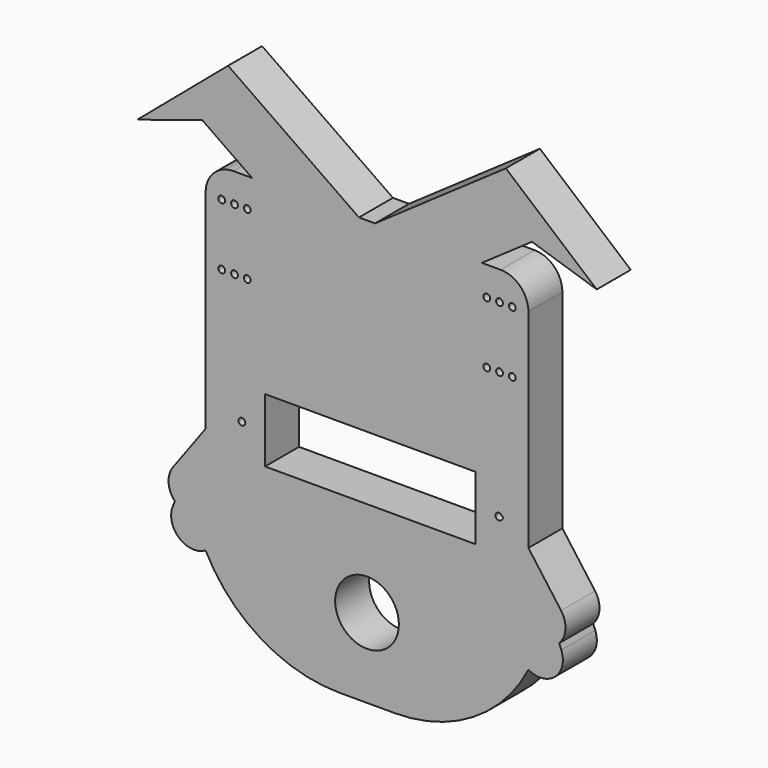
from build123d import *

# Parameters (mm, degrees)
F0_R        = 15
F0_R_2      = 1.6
F1_DEPTH    = 20
F2_R        = 11.6045153918
F3_DEPTH    = 20
F4_T1_DEPTH = 334.7254047122
F6_R        = 13.1169251871
F7_T1_DEPTH = 119.353153646
F7_T3_DEPTH = 204.1085089788


# Not quite as in the source:
# - a fillet or chamfer that OpenCascade refuses, or shapes differently, is made with other operations: its cross-section is extruded or revolved along the edge and cut away or added


with BuildPart() as f1:
    # F0 (on Front) → F1 (new body)
    with BuildSketch(Plane.XZ):
        Polygon((-54.1030839086, 102.6), (-76.0052064898, 102.6), (-76.0052064898, -8.4487323015), (-76.0052064898, -58.9213789776), (-76.0052064898, -97.4), (75.9947935102, -97.4), (75.9947935102, -58.9213789776), (75.9947935102, -8.4487323015), (75.9947935102, 102.6), (54.0926709289, 102.6), (3.7848638975, 102.6), (-0.0052064898, 102.6), (-3.7952768771, 102.6), align=None)
        with Locations((0, -60)):
            Circle(F0_R, mode=Mode.SUBTRACT)
        Polygon((-48.0052064898, 15), (-0.0052064898, 15), (50.9947935102, 15), (63.2902167228, 1.058300535), (64.2235500655, 0), (63.2902167424, -1.0583005129), (50.9947935102, -15), (-48.0052064898, -15), (-61.2339630452, 0), align=None, mode=Mode.SUBTRACT)
        with Locations((-68.4052064898, 60)):
            Circle(F0_R_2, mode=Mode.SUBTRACT)
        with Locations((-62.4052064898, 60)):
            Circle(F0_R_2, mode=Mode.SUBTRACT)
        with Locations((-56.4052064898, 60)):
            Circle(F0_R_2, mode=Mode.SUBTRACT)
        with Locations((-68.4052064898, 89)):
            Circle(F0_R_2, mode=Mode.SUBTRACT)
        with Locations((-62.4052064898, 89)):
            Circle(F0_R_2, mode=Mode.SUBTRACT)
        with Locations((-56.4052064898, 89)):
            Circle(F0_R_2, mode=Mode.SUBTRACT)
        with Locations((56.3947935102, 60)):
            Circle(F0_R_2, mode=Mode.SUBTRACT)
        with Locations((62.3947935102, 60)):
            Circle(F0_R_2, mode=Mode.SUBTRACT)
        with Locations((68.3947935102, 60)):
            Circle(F0_R_2, mode=Mode.SUBTRACT)
        with Locations((56.3947935102, 89)):
            Circle(F0_R_2, mode=Mode.SUBTRACT)
        with Locations((62.3947935102, 89)):
            Circle(F0_R_2, mode=Mode.SUBTRACT)
        with Locations((68.3947935102, 89)):
            Circle(F0_R_2, mode=Mode.SUBTRACT)
        Polygon((-77.668659389, 119.0051808953), (-54.1030839086, 102.6), (-3.7952768771, 102.6), (-65.412312746, 145.4675197601), (-108.1871464849, 109.1671809554), align=None)
        Polygon((-76.0052064898, -58.9213789776), (-76.0052064898, -8.4487323015), (-103.1352177745, -45.4250201583), (-90.5148283129, -43.2038009167), (-105.0179273372, -79.8825249076), align=None)
        Polygon((65.4018997664, 145.4675197601), (3.7848638975, 102.6), (54.0926709289, 102.6), (77.6582464094, 119.0051808953), (108.1767335052, 109.1671809554), align=None)
        Polygon((75.9947935102, -8.4487323015), (75.9947935102, -58.9213789776), (105.0075143576, -79.8825249076), (90.5044153333, -43.2038009167), (103.1248047948, -45.4250201583), align=None)
        with BuildLine():
            Line((63.2902167228, 1.058300535), (50.9947935102, 15))
            Line((50.9947935102, 15), (50.9947935102, -15))
            Line((50.9947935102, -15), (63.2902167424, -1.0583005129))
            ThreePointArc((63.2902167424, -1.0583005129), (60.4902167322, -1.48e-08), (63.2902167228, 1.058300535))
        make_face()
        Polygon((-48.0052064898, -15), (-48.0052064898, 15), (-61.2339630452, 0), align=None)
        with Locations((-58.9281324463, 0)):
            Circle(F0_R_2, mode=Mode.SUBTRACT)
    extrude(amount=F1_DEPTH)

    # F2
    f2_edges = [f1.edges().sort_by_distance(p)[0] for p in [
        (-76.005206, -10, 102.6),
        (-76.005206, -10, -97.4),
        (75.994794, -10, -97.4),
        (75.994794, -10, 102.6),
    ]]
    fillet(f2_edges, radius=F2_R)

    # F0 (on Front) → F3 (join)
    with BuildSketch(Plane.XZ):
        Polygon((-54.1030839086, 102.6), (-76.0052064898, 102.6), (-76.0052064898, -8.4487323015), (-76.0052064898, -58.9213789776), (-76.0052064898, -97.4), (75.9947935102, -97.4), (75.9947935102, -58.9213789776), (75.9947935102, -8.4487323015), (75.9947935102, 102.6), (54.0926709289, 102.6), (3.7848638975, 102.6), (-0.0052064898, 102.6), (-3.7952768771, 102.6), align=None)
        with Locations((0, -60)):
            Circle(F0_R, mode=Mode.SUBTRACT)
        Polygon((-48.0052064898, 15), (-0.0052064898, 15), (50.9947935102, 15), (63.2902167228, 1.058300535), (64.2235500655, 0), (63.2902167424, -1.0583005129), (50.9947935102, -15), (-48.0052064898, -15), (-61.2339630452, 0), align=None, mode=Mode.SUBTRACT)
        with Locations((-68.4052064898, 60)):
            Circle(F0_R_2, mode=Mode.SUBTRACT)
        with Locations((-62.4052064898, 60)):
            Circle(F0_R_2, mode=Mode.SUBTRACT)
        with Locations((-56.4052064898, 60)):
            Circle(F0_R_2, mode=Mode.SUBTRACT)
        with Locations((-68.4052064898, 89)):
            Circle(F0_R_2, mode=Mode.SUBTRACT)
        with Locations((-62.4052064898, 89)):
            Circle(F0_R_2, mode=Mode.SUBTRACT)
        with Locations((-56.4052064898, 89)):
            Circle(F0_R_2, mode=Mode.SUBTRACT)
        with Locations((56.3947935102, 60)):
            Circle(F0_R_2, mode=Mode.SUBTRACT)
        with Locations((62.3947935102, 60)):
            Circle(F0_R_2, mode=Mode.SUBTRACT)
        with Locations((68.3947935102, 60)):
            Circle(F0_R_2, mode=Mode.SUBTRACT)
        with Locations((56.3947935102, 89)):
            Circle(F0_R_2, mode=Mode.SUBTRACT)
        with Locations((62.3947935102, 89)):
            Circle(F0_R_2, mode=Mode.SUBTRACT)
        with Locations((68.3947935102, 89)):
            Circle(F0_R_2, mode=Mode.SUBTRACT)
        Polygon((-77.668659389, 119.0051808953), (-54.1030839086, 102.6), (-3.7952768771, 102.6), (-65.412312746, 145.4675197601), (-108.1871464849, 109.1671809554), align=None)
        Polygon((-76.0052064898, -58.9213789776), (-76.0052064898, -8.4487323015), (-103.1352177745, -45.4250201583), (-90.5148283129, -43.2038009167), (-105.0179273372, -79.8825249076), align=None)
        Polygon((65.4018997664, 145.4675197601), (3.7848638975, 102.6), (54.0926709289, 102.6), (77.6582464094, 119.0051808953), (108.1767335052, 109.1671809554), align=None)
        Polygon((75.9947935102, -8.4487323015), (75.9947935102, -58.9213789776), (105.0075143576, -79.8825249076), (90.5044153333, -43.2038009167), (103.1248047948, -45.4250201583), align=None)
        Polygon((-48.0052064898, -15), (-48.0052064898, 15), (-61.2339630452, 0), align=None)
        with Locations((-58.9281324463, 0)):
            Circle(F0_R_2, mode=Mode.SUBTRACT)
        with BuildLine():
            Line((63.2902167228, 1.058300535), (50.9947935102, 15))
            Line((50.9947935102, 15), (50.9947935102, -15))
            Line((50.9947935102, -15), (63.2902167424, -1.0583005129))
            ThreePointArc((63.2902167424, -1.0583005129), (60.4902167322, -1.48e-08), (63.2902167228, 1.058300535))
        make_face()
    extrude(amount=F3_DEPTH)

    # F4: fillet of radius 70.723525766 on 2 edges, made by hand

    # F4_s2 → F4_t1 (cut)
    with BuildSketch(Plane.XZ.offset(-157.3627023561)):
        with BuildLine():
            ThreePointArc((-76.0052064898, -58.9213789776), (-49.9474116045, -87.018376956), (-13.0601255474, -97.4))
            Line((-13.0601255474, -97.4), (-76.0052064898, -97.4))
            Line((-76.0052064898, -97.4), (-76.0052064898, -58.9213789776))
        make_face()
        with BuildLine():
            ThreePointArc((13.0497125677, -97.4), (49.9369986248, -87.018376956), (75.9947935102, -58.9213789776))
            Line((75.9947935102, -58.9213789776), (75.9947935102, -97.4))
            Line((75.9947935102, -97.4), (13.0497125677, -97.4))
        make_face()
    extrude(amount=F4_T1_DEPTH, mode=Mode.SUBTRACT)

    # F6
    f6_edges = [f1.edges().sort_by_distance(p)[0] for p in [
        (75.994794, -10, 102.6),
        (-76.005206, -10, 102.6),
    ]]
    fillet(f6_edges, radius=F6_R)

    # F7: fillet of radius 10.7873299095 on 4 edges, made by hand

    # F7_s2 → F7_t1 (cut)
    with BuildSketch(Plane.XZ.offset(-49.676576823)):
        with BuildLine():
            ThreePointArc((91.3700727829, -29.4041512397), (93.4388619061, -36.4609035493), (90.5044153333, -43.2038009167))
            Line((90.5044153333, -43.2038009167), (103.1248047948, -45.4250201583))
            Line((103.1248047948, -45.4250201583), (91.3700727829, -29.4041512397))
        make_face()
        with BuildLine():
            ThreePointArc((-90.5148283129, -43.2038009167), (-93.4492748858, -36.4609035493), (-91.3804857626, -29.4041512397))
            Line((-91.3804857626, -29.4041512397), (-103.1352177745, -45.4250201583))
            Line((-103.1352177745, -45.4250201583), (-90.5148283129, -43.2038009167))
        make_face()
    extrude(amount=F7_T1_DEPTH, mode=Mode.SUBTRACT)

    # F7_s4 → F7_t3 (cut)
    with BuildSketch(Plane.XZ.offset(-92.0542544894)):
        with BuildLine():
            ThreePointArc((-76.0052064898, -58.9213789776), (-88.4725874625, -57.7926608942), (-91.4783185714, -45.6404934608))
            Line((-91.4783185714, -45.6404934608), (-105.0179273372, -79.8825249076))
            Line((-105.0179273372, -79.8825249076), (-76.0052064898, -58.9213789776))
        make_face()
        with BuildLine():
            ThreePointArc((91.4679055918, -45.6404934608), (88.4621744828, -57.7926608942), (75.9947935102, -58.9213789776))
            Line((75.9947935102, -58.9213789776), (105.0075143576, -79.8825249076))
            Line((105.0075143576, -79.8825249076), (91.4679055918, -45.6404934608))
        make_face()
    extrude(amount=F7_T3_DEPTH, mode=Mode.SUBTRACT)


solid = f1.part
